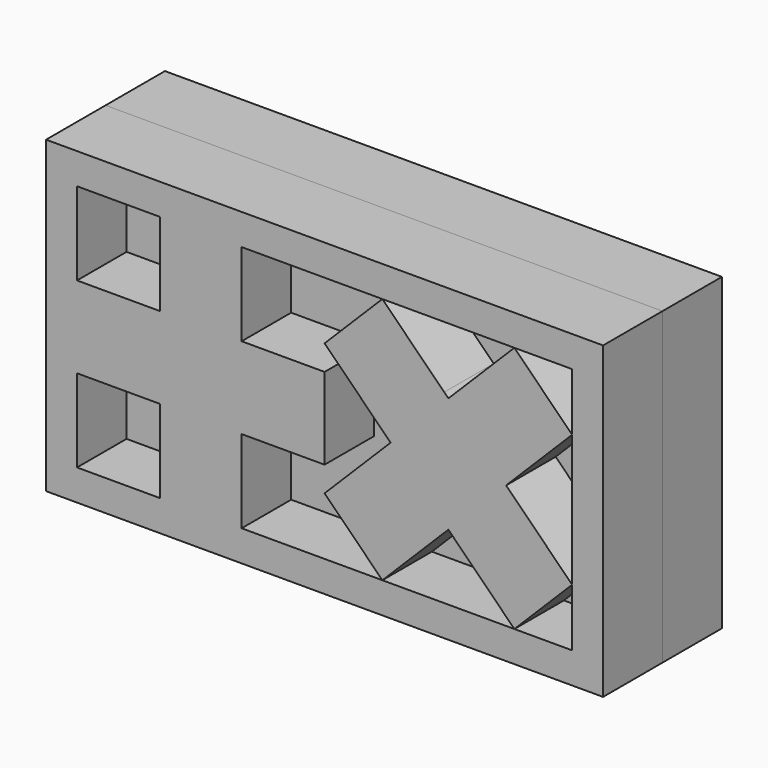
from build123d import *

# Parameters (mm, degrees)
F0_W     = 45
F0_H     = 25
F1_DEPTH = 1
F2_W     = 45
F2_H     = 25
F3_DEPTH = 5
F4_DEPTH = 5
F5_DEPTH = 5


# Not quite as in the source:
# - ends of sketch curves that miss each other by under 0.0002 mm in the source are joined


with BuildPart() as f1:
    # F0 (on Front) → F1 (new body)
    with BuildSketch(Plane.XZ):
        Rectangle(F0_W, F0_H)
    extrude(amount=F1_DEPTH)

    # F2 (on face) → F3 (join)
    with BuildSketch(Plane.XZ.offset(1)):
        Rectangle(F2_W, F2_H)
        Polygon((-20, 3.3), (-20, 10), (-13.3, 10), (-6.7, 10), (4.6669047558, 10), (15.3330952385, 10), (20, 10), (20, 5.3330952385), (20, -5.3329034452), (20, -10), (15.3329034452, -10), (4.6669112521, -10), (-6.7, -10), (-13.3, -10), (-20, -10), (-20, -3.3), align=None, mode=Mode.SUBTRACT)
    extrude(amount=F3_DEPTH)

    # F2 (on face) → F4 (join)
    with BuildSketch(Plane.XZ.offset(1)):
        Polygon((-6.7, 10), (-13.3, 10), (-13.3, 3.3), (-20, 3.3), (-20, -3.3), (-13.3, -3.3), (-13.3, -10), (-6.7, -10), (-6.7, -3.3), (0, -3.3), (0, 0), (0, 3.3), (-6.7, 3.3), align=None)
    extrude(amount=F4_DEPTH)


with BuildPart() as f5:
    # F2 (on face) → F5 (new body)
    with BuildSketch(Plane.XZ.offset(1)):
        Polygon((9.6650526696, 5.0018520863), (4.6669047558, 10), (0, 5.3330952442), (4.9981479137, 0.3349473304), (5.3329483647, -0.0001468775), (1.29926e-05, -5.3330822516), (4.6669047558, -10), (9.9999041025, -4.6670006553), (15.3329034452, -10), (20, -5.3329034452), (14.6669047548, -4.7e-09), (20, 5.3330952385), (15.3330952385, 10), (9.9999999982, 4.6669047577), align=None)
    extrude(amount=F5_DEPTH)


with BuildPart() as f6_1:
    # F6: instance of F1
    add(f1.part.mirror(Plane.XZ))


with BuildPart() as f6_2:
    # F6: instance of F5
    add(f5.part.mirror(Plane.XZ))


solid = Compound([f1.part, f5.part, f6_1.part, f6_2.part])
